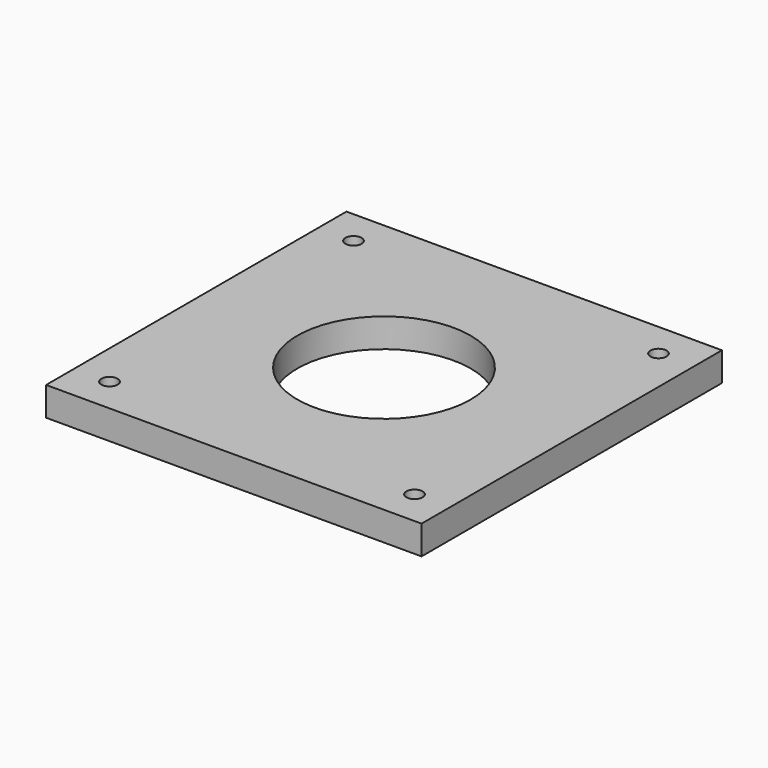
from build123d import *

# Parameters (mm, degrees)
F0_W     = 82.55
F0_H     = 82.55
F0_R     = 1.778
F0_R_2   = 19.05
F1_DEPTH = 6.35


# Not quite as in the source:
# - a length typed as a fraction of an inch, garbled in the dataset ("3 / 203.2 mm" for 3/8 in), is restored


with BuildPart() as f1:
    # F0 (on Top) → F1 (new body)
    with BuildSketch(Plane.XY):
        Rectangle(F0_W, F0_H)
        with Locations((-33.528, -33.528)):
            Circle(F0_R, mode=Mode.SUBTRACT)
        with Locations((33.528, -33.528)):
            Circle(F0_R, mode=Mode.SUBTRACT)
        with Locations((-33.528, 33.528)):
            Circle(F0_R, mode=Mode.SUBTRACT)
        Circle(F0_R_2, mode=Mode.SUBTRACT)
        with Locations((33.528, 33.528)):
            Circle(F0_R, mode=Mode.SUBTRACT)
    extrude(amount=F1_DEPTH)


solid = f1.part
